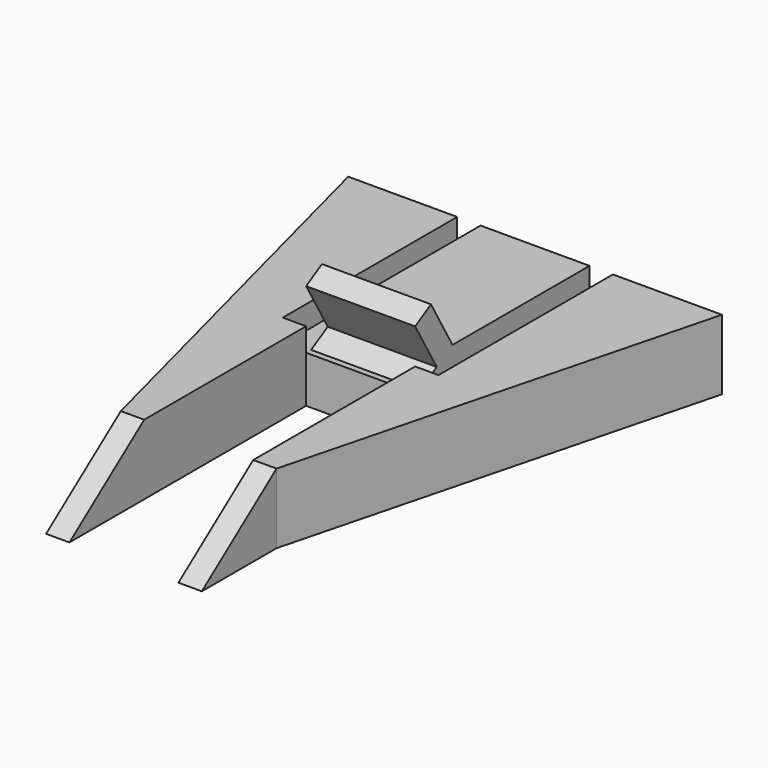
from build123d import *

# Parameters (mm, degrees)
F1_DEPTH      = 3.81
F1_DEPTH_BACK = 7.62
F0_W          = 3.81
F0_H          = 17.78
F2_DEPTH      = 7.62
F3_W          = 17.78
F3_H          = 7.62
F4_DEPTH      = 7.62
F6_DEPTH      = 17.78
F7_W          = 17.78
F7_H          = 11.43
F8_DEPTH      = 33.02
F9_DEPTH      = 17.78
F10_W         = 3.81
F10_H         = 11.43
F11_DEPTH     = 15.24
F12_W         = 3.81
F12_H         = 11.43
F13_DEPTH     = 15.24
F15_DEPTH     = 25.4
F18_DEPTH     = 25.4


# Not quite as in the source:
# - a feature names something its author has since deleted; it is built from what else it names


with BuildPart() as f1:
    # F0 (on Top) → F1 (new body, two sides)
    with BuildSketch(Plane.XY) as f1_sk:
        Polygon((-54.4414605618, -0.1530551207), (-79.8414605618, -0.1530551207), (-79.8414605618, -50.9530551207), (-3.6414605618, -50.9530551207), (-3.6414605618, -0.1530551207), (-29.0414605618, -0.1530551207), (-29.0414605618, -17.9330551207), (-32.8514605618, -17.9330551207), (-32.8514605618, -0.1530551207), (-50.6314605618, -0.1530551207), (-50.6314605618, -17.9330551207), (-54.4414605618, -17.9330551207), align=None)
    extrude(amount=F1_DEPTH)
    extrude(f1_sk.sketch, amount=-F1_DEPTH_BACK)

    # F0 (on Top) → F2 (join)
    with BuildSketch(Plane.XY):
        with Locations((-52.5364605618, -9.0430551207)):
            Rectangle(F0_W, F0_H)
        with Locations((-30.9464605618, -9.0430551207)):
            Rectangle(F0_W, F0_H)
    extrude(amount=-F2_DEPTH)

    # F3 (on face) → F4 (join)
    with BuildSketch(Plane.XY.offset(3.81)):
        with Locations((-41.7414605618, -14.1230551207)):
            Rectangle(F3_W, F3_H)
    extrude(amount=F4_DEPTH)

    # F5 (on face) → F6 (cut)
    with BuildSketch(Plane.YZ.offset(-32.8514605618)):
        Polygon((-14.7124641719, 11.43), (-10.3130551207, 3.81), (-10.3130551207, 11.43), align=None)
        Polygon((-17.9330551207, 9.5705909488), (-14.7124641719, 11.43), (-17.9330551207, 11.43), align=None)
        Polygon((-16.9121686975, 0), (-13.5336460694, 1.9505909488), (-17.9330551207, 9.5705909488), (-17.9330551207, 3.81), (-17.9330551207, 0), align=None)
    extrude(amount=-F6_DEPTH, mode=Mode.SUBTRACT)

    # F7 (on face) → F8 (cut)
    with BuildSketch(Plane.XZ.offset(50.9530551207)):
        with Locations((-41.7414605618, -1.905)):
            Rectangle(F7_W, F7_H)
    extrude(amount=-F8_DEPTH, mode=Mode.SUBTRACT)

    # F9 (add): a face of the model
    f9_faces = [f1.faces().sort_by_distance(p)[0] for p in [
        (-41.7414605618, -0.1530551207, -2.0363793103),
    ]]
    extrude(f9_faces, amount=F9_DEPTH)

    # F10 (on face) → F11 (join)
    with BuildSketch(Plane.XZ.offset(50.9530551207)):
        with Locations((-52.5364605618, -1.905)):
            Rectangle(F10_W, F10_H)
    extrude(amount=F11_DEPTH)

    # F12 (on face) → F13 (join)
    with BuildSketch(Plane.XZ.offset(50.9530551207)):
        with Locations((-30.9464605618, -1.905)):
            Rectangle(F12_W, F12_H)
    extrude(amount=F13_DEPTH)

    # F14 (on face) → F15 (cut)
    with BuildSketch(Plane(origin=(-54.4414605618, 0, 0), x_dir=(0, -1, 0), z_dir=(-1, 0, 0))):
        Polygon((66.1930551207, 3.81), (50.9530551207, 3.81), (66.1930551207, -7.62), align=None)
    extrude(amount=-F15_DEPTH, mode=Mode.SUBTRACT)

    # F16 (on face) + F17 (on face) → F18 (cut)
    with BuildSketch(Plane.XY.offset(3.81)):
        Polygon((-54.4414605618, -50.9530551207), (-72.2214605618, 17.6269448793), (-79.8414605618, 17.6269448793), (-79.8414605618, -50.9530551207), align=None)
    with BuildSketch(Plane.XY.offset(3.81)):
        Polygon((-3.6414605618, 17.6269448793), (-11.2614605618, 17.6269448793), (-29.0414605618, -50.9530551207), (-3.6414605618, -50.9530551207), align=None)
    extrude(amount=-F18_DEPTH, mode=Mode.SUBTRACT)


solid = f1.part
